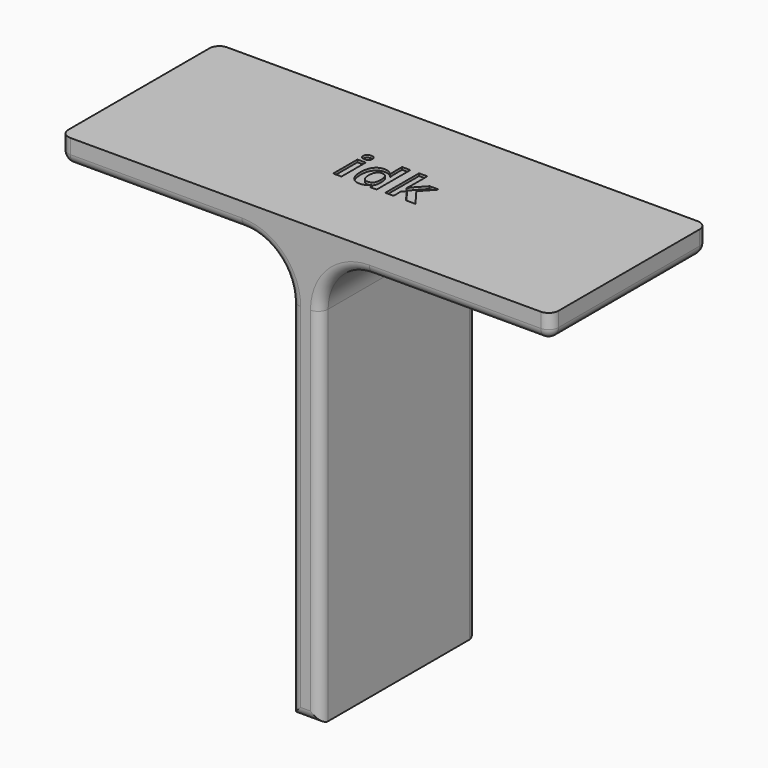
from build123d import *

# Parameters (mm, degrees)
F0_W         = 47
F0_H         = 40
F0_W_2       = 6
F1_DEPTH     = 5
F2_DEPTH     = 84
F3_R         = 10
F4_R         = 2
F5_TEXT_SIZE = 11.3325647449
F6_DEPTH     = 0.5


# Not quite as in the source:
# - Text() gives the source's letters only with a copy of the font that has no kerning and outlines rounded to 1/6400 em; it was checked with that copy


with BuildPart() as f1:
    # F0 (on Top) → F1 (new body)
    with BuildSketch(Plane.XY):
        with Locations((-26.5, 0)):
            Rectangle(F0_W, F0_H)
        Rectangle(F0_W_2, F0_H)
        with Locations((26.5, 0)):
            Rectangle(F0_W, F0_H)
    extrude(amount=F1_DEPTH)

    # F0 (on Top) → F2 (join)
    with BuildSketch(Plane.XY):
        Rectangle(F0_W_2, F0_H)
    extrude(amount=-F2_DEPTH)

    # F3
    f3_edges = [f1.edges().sort_by_distance(p)[0] for p in [
        (3, 0, 0),
        (-3, 0, 0),
    ]]
    fillet(f3_edges, radius=F3_R)

    # F4
    f4_edges = [f1.edges().sort_by_distance(p)[0] for p in [
        (-50, 0, 0),
        (-31.5, 20, 0),
        (-50, 20, 2.5),
        (31.5, 20, 0),
        (-31.5, -20, 0),
        (-50, -20, 2.5),
        (31.5, -20, 0),
        (50, -20, 2.5),
        (50, 0, 0),
        (50, 20, 2.5),
        (0, 20, -84),
        (0, -20, -84),
    ]]
    fillet(f4_edges, radius=F4_R)

    # F5 (on face) → F6 (cut)
    with BuildSketch(Plane.XY.offset(5)):
        with Locations((-8.5013269563, -3.4363170125)):
            Text('idk', F5_TEXT_SIZE, font='Open Sans', font_style=FontStyle.BOLD, text_align=(TextAlign.LEFT, TextAlign.BOTTOM))
    extrude(amount=-F6_DEPTH, mode=Mode.SUBTRACT)


solid = f1.part
